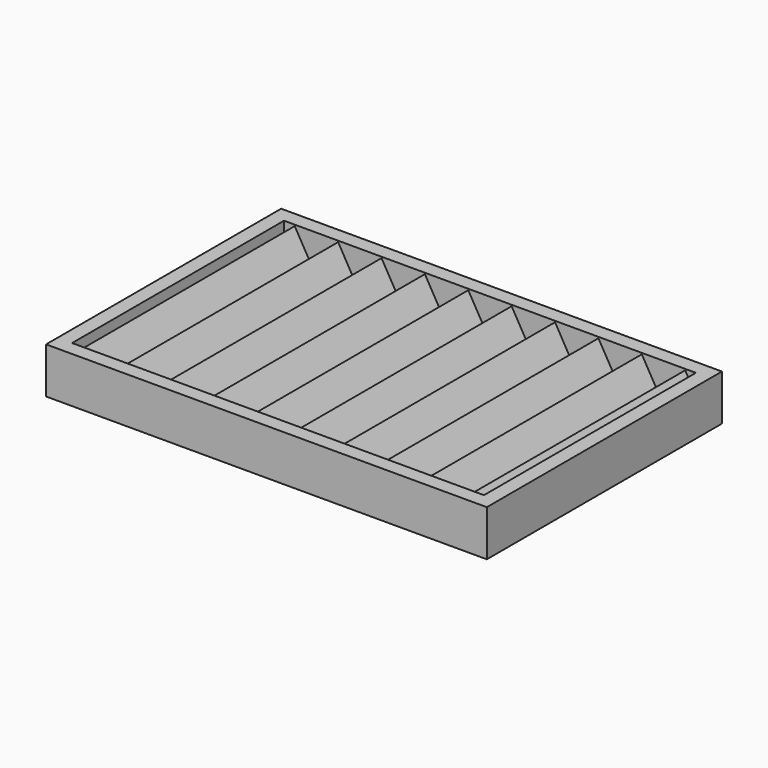
from build123d import *

# Parameters (mm, degrees)
F1_DEPTH = 50
F2_W     = 152.4
F2_H     = 101.6
F2_W_2   = 142.4
F2_H_2   = 91.6
F3_DEPTH = 7.9375


# Not quite as in the source:
# - a length typed as a fraction of an inch, garbled in the dataset ("3 / 203.2 mm" for 3/8 in), is restored
# - a feature names something its author has since deleted; it is built from what else it names


with BuildPart() as f1:
    # F0 (on Front) → F1 (new body, symmetric)
    with BuildSketch(Plane.XZ):
        Polygon((-67.5, 7.5), (-75, -5.4990042023), (-75, -7.5), (-67.5, 5.4990042023), (-60, -7.5), (-52.5, 5.4990042023), (-45, -7.5), (-37.5, 5.4990042023), (-30, -7.5), (-22.5, 5.4990042023), (-15, -7.5), (-7.5, 5.4990042023), (0, -7.5), (7.5, 5.4990042023), (15, -7.5), (22.5, 5.4990042023), (30, -7.5), (37.5, 5.4990042023), (45, -7.5), (52.5, 5.4990042023), (60, -7.5), (67.5, 5.4990042023), (75, -7.5), (75, -5.4990042023), (67.5, 7.5), (60, -5.4990042023), (52.5, 7.5), (45, -5.4990042023), (37.5, 7.5), (30, -5.4990042023), (22.5, 7.5), (15, -5.4990042023), (7.5, 7.5), (0, -5.4990042023), (-7.5, 7.5), (-15, -5.4990042023), (-22.5, 7.5), (-30, -5.4990042023), (-37.5, 7.5), (-45, -5.4990042023), (-52.5, 7.5), (-60, -5.4990042023), align=None)
    extrude(amount=F1_DEPTH, both=True)


with BuildPart() as f3:
    # F2 (on Top) → F3 (new body, symmetric)
    with BuildSketch(Plane.XY):
        Rectangle(F2_W, F2_H)
        Rectangle(F2_W_2, F2_H_2, mode=Mode.SUBTRACT)
    extrude(amount=F3_DEPTH, both=True)


solid = Compound([f1.part, f3.part])
